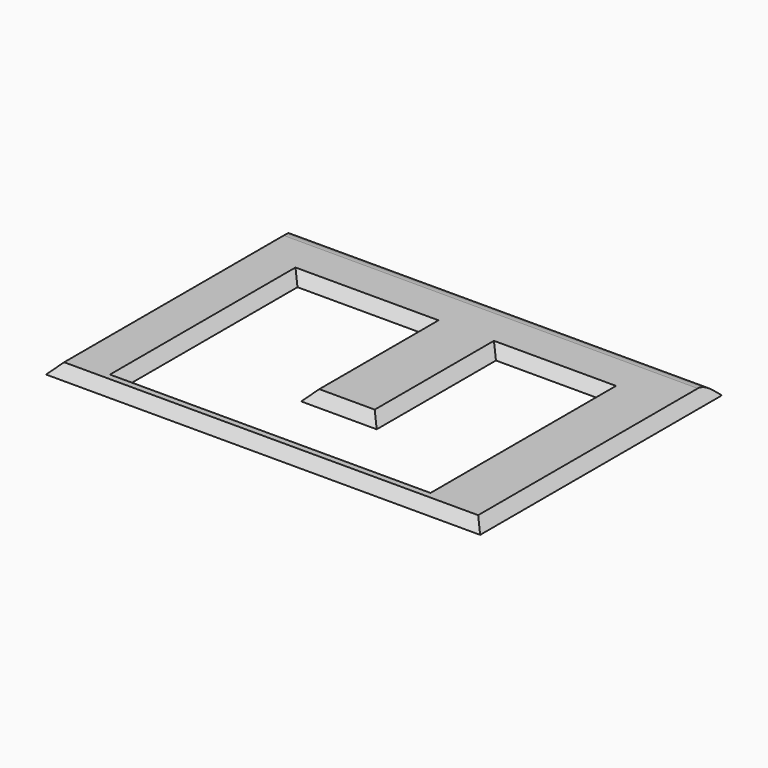
from build123d import *

# Parameters (mm, degrees)
F0_W         = 124.8456425965
F0_H         = 88.3170031011
F1_DEPTH     = 2.7760323137
F2_T1_DEPTH  = 114.4453022588
F3_T1_DEPTH  = 145.8939417542
F4_T1_DEPTH  = 109.3653022588
F5_T1_DEPTH  = 140.8139417542
F6_R         = 5.08
F7_T1_DEPTH  = 56.8432509899
F8_T1_DEPTH  = 23.6501246691
F9_T4_DEPTH  = 47.6030598057
F10_T4_DEPTH = 72.4922642685
F11_T4_DEPTH = 72.4922642685
F12_T4_DEPTH = 74.9874005688
F13_T1_DEPTH = 41.4855244232
F14_T4_DEPTH = 109.3624946917


# Not quite as in the source:
# - a fillet or chamfer that OpenCascade refuses, or shapes differently, is made with other operations: its cross-section is extruded or revolved along the edge and cut away or added


with BuildPart() as f1:
    # F0 (on Top) → F1 (new body)
    with BuildSketch(Plane.XY):
        with Locations((2.7440618724, 2.717172727)):
            Rectangle(F0_W, F0_H)
        Polygon((-38.1721407175, -32.3632955551), (-38.1721407175, 24.4799554348), (-8.7132304907, 24.4799554348), (-8.7132304907, -16.804009676), (16.8039947748, -16.804009676), (16.8039947748, 24.4799554348), (40.4541194439, 24.4799554348), (40.4541194439, -32.3632955551), align=None, mode=Mode.SUBTRACT)
    extrude(amount=F1_DEPTH)

    # F2: chamfer of 5.08 on 1 edges, made by hand

    # F2_s2 → F2_t1 (cut)
    with BuildSketch(Plane.XZ.offset(-59.9398238564)):
        Polygon((65.1668831706, -2.3039676863), (60.0868831706, 2.7760323137), (65.1668831706, 2.7760323137), align=None)
    extrude(amount=F2_T1_DEPTH, mode=Mode.SUBTRACT)

    # F3: chamfer of 5.08 on 1 edges, made by hand

    # F3_s2 → F3_t1 (cut)
    with BuildSketch(Plane.YZ.offset(-72.7429090047)):
        Polygon((46.8756742775, -2.3039676863), (41.7956742775, 2.7760323137), (46.8756742775, 2.7760323137), align=None)
    extrude(amount=F3_T1_DEPTH, mode=Mode.SUBTRACT)

    # F4: chamfer of 5.08 on 1 edges, made by hand

    # F4_s2 → F4_t1 (cut)
    with BuildSketch(Plane.XZ.offset(-54.8598238564)):
        Polygon((-59.6787594259, -2.3039676863), (-54.5987594259, 2.7760323137), (-59.6787594259, 2.7760323137), align=None)
    extrude(amount=F4_T1_DEPTH, mode=Mode.SUBTRACT)

    # F5: chamfer of 5.08 on 1 edges, made by hand

    # F5_s2 → F5_t1 (cut)
    with BuildSketch(Plane.YZ.offset(-67.6629090048)):
        Polygon((-41.4413288236, -2.3039676863), (-36.3613288236, 2.7760323137), (-41.4413288236, 2.7760323137), align=None)
    extrude(amount=F5_T1_DEPTH, mode=Mode.SUBTRACT)

    # F6
    f6_edges = [f1.edges().sort_by_distance(p)[0] for p in [
        (2.744062, 41.795674, 2.776032),
    ]]
    fillet(f6_edges, radius=F6_R)

    # F7: chamfer of 5.08 on 1 edges, made by hand

    # F7_s2 → F7_t1 (cut)
    with BuildSketch(Plane.XZ.offset(-24.4799554348)):
        Polygon((-43.2521407175, 2.7760323137), (-38.1721407175, -2.3039676863), (-38.1721407175, 2.7760323137), align=None)
    extrude(amount=F7_T1_DEPTH, mode=Mode.SUBTRACT)

    # F8: chamfer of 5.08 on 1 edges, made by hand

    # F8_s2 → F8_t1 (cut)
    with BuildSketch(Plane.YZ.offset(16.8039947748)):
        Polygon((24.4799554348, -2.3039676863), (29.5599554348, 2.7760323137), (24.4799554348, 2.7760323137), align=None)
    extrude(amount=F8_T1_DEPTH, mode=Mode.SUBTRACT)

    # F9: chamfer of 5.08 on 1 edges, made by hand


with BuildPart() as f9_tool2:
    # F9_s3 → F9_t4 (new body)
    with BuildSketch(Plane.YZ.offset(-56.3162902964)):
        Polygon((24.4799554348, -2.3039676863), (29.5599554348, 2.7760323137), (24.4799554348, 2.7760323137), align=None)
    extrude(amount=F9_T4_DEPTH)

    split(bisect_by=Plane(origin=(-20.2380542019, 0, -20.2380542019), x_dir=(0, 1, 0), z_dir=(0.7071067812, 0, 0.7071067812)), keep=Keep.TOP)


with BuildPart() as f1_1:
    add(f1.part)

    # F9_t1: cut F9_tool2
    add(f9_tool2.part, mode=Mode.SUBTRACT)

    # F10: chamfer of 5.08 on 1 edges, made by hand


with BuildPart() as f10_tool2:
    # F10_s3 → F10_t4 (new body)
    with BuildSketch(Plane.XZ.offset(-42.6241050137)):
        Polygon((-8.7132304907, -2.3039676863), (-3.6332304907, 2.7760323137), (-8.7132304907, 2.7760323137), align=None)
    extrude(amount=F10_T4_DEPTH)

    split(bisect_by=Plane(origin=(0, 13.3919615606, -13.3919615605), x_dir=(1, 0, 0), z_dir=(0, -0.7071067812, 0.7071067812)), keep=Keep.TOP)


with BuildPart() as f1_2:
    add(f1_1.part)

    # F10_t1: cut F10_tool2
    add(f10_tool2.part, mode=Mode.SUBTRACT)

    # F11: chamfer of 5.08 on 1 edges, made by hand


with BuildPart() as f11_tool2:
    # F11_s3 → F11_t4 (new body)
    with BuildSketch(Plane.XZ.offset(29.8681592548)):
        Polygon((16.8039947748, -2.3039676863), (11.7239947748, 2.7760323137), (16.8039947748, 2.7760323137), align=None)
    extrude(amount=-F11_T4_DEPTH)

    split(bisect_by=Plane(origin=(0, 13.3919615606, -13.3919615606), x_dir=(1, 0, 0), z_dir=(0, -0.7071067812, 0.7071067812)), keep=Keep.TOP)


with BuildPart() as f1_3:
    add(f1_2.part)

    # F11_t1: cut F11_tool2
    add(f11_tool2.part, mode=Mode.SUBTRACT)

    # F12: chamfer of 5.08 on 1 edges, made by hand


with BuildPart() as f12_tool2:
    # F12_s3 → F12_t4 (new body)
    with BuildSketch(Plane.XZ.offset(-42.6241050137)):
        Polygon((40.4541194439, -2.3039676863), (45.5341194439, 2.7760323137), (40.4541194439, 2.7760323137), align=None)
    extrude(amount=F12_T4_DEPTH)

    split(bisect_by=Plane(origin=(0, 13.3919615606, -13.3919615606), x_dir=(1, 0, 0), z_dir=(0, -0.7071067812, 0.7071067812)), keep=Keep.TOP)


with BuildPart() as f1_4:
    add(f1_3.part)

    # F12_t1: cut F12_tool2
    add(f12_tool2.part, mode=Mode.SUBTRACT)

    # F13: chamfer of 5.08 on 1 edges, made by hand

    # F13_s2 → F13_t1 (cut)
    with BuildSketch(Plane.YZ.offset(-16.6973800696)):
        Polygon((-16.804009676, -2.3039676863), (-11.724009676, 2.7760323137), (-16.804009676, 2.7760323137), align=None)
    extrude(amount=F13_T1_DEPTH, mode=Mode.SUBTRACT)

    # F14: chamfer of 5.08 on 1 edges, made by hand


with BuildPart() as f14_tool2:
    # F14_s3 → F14_t4 (new body)
    with BuildSketch(Plane.YZ.offset(-53.5402579827)):
        Polygon((-37.4432955551, 0), (-32.3632955551, 5.08), (-32.3632955551, 0), align=None)
    extrude(amount=F14_T4_DEPTH)

    split(bisect_by=Plane(origin=(-20.2380542019, 0, -20.2380542019), x_dir=(0, 1, 0), z_dir=(0.7071067812, 0, 0.7071067812)), keep=Keep.TOP)

    split(bisect_by=Plane(origin=(21.3790435651, 0, -21.3790435651), x_dir=(0, 1, 0), z_dir=(-0.7071067812, 0, 0.7071067812)), keep=Keep.TOP)


with BuildPart() as f1_5:
    add(f1_4.part)

    # F14_t1: cut F14_tool2
    add(f14_tool2.part, mode=Mode.SUBTRACT)


solid = f1_5.part
